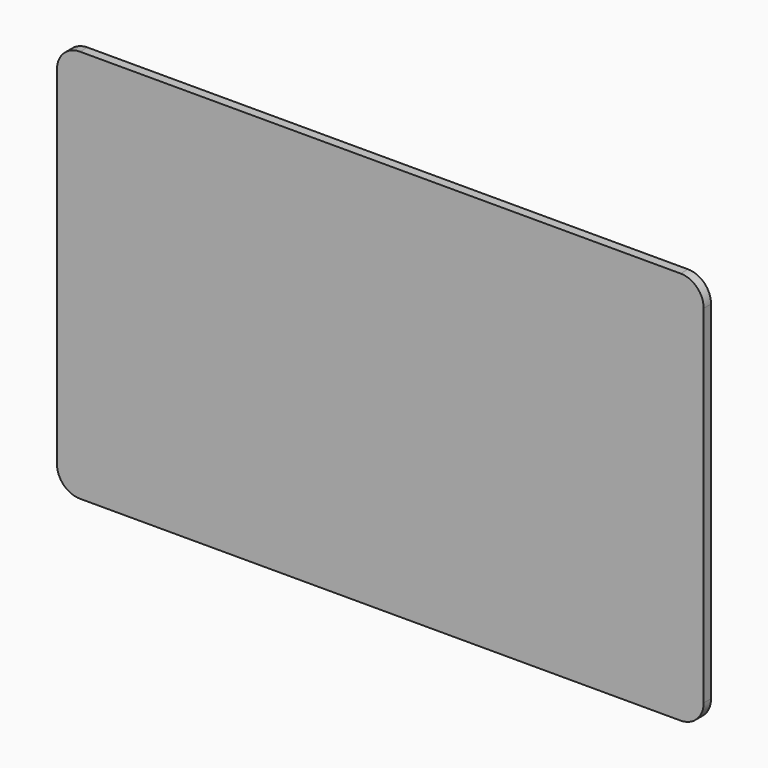
from build123d import *

# Parameters (mm, degrees)
F1_DEPTH = 3


# Not quite as in the source:
# - a feature names something its author has since deleted; it is built from what else it names


with BuildPart() as f1:
    # F0 (on Front) → F1 (new body)
    with BuildSketch(Plane.XZ):
        with BuildLine():
            ThreePointArc((105, 56.4), (102.8033008589, 61.7033008589), (97.5, 63.9))
            Line((97.5, 63.9), (-97.5, 63.9))
            ThreePointArc((-97.5, 63.9), (-102.8033008589, 61.7033008589), (-105, 56.4))
            Line((-105, 56.4), (-105, -56.4))
            ThreePointArc((-105, -56.4), (-102.8033008589, -61.7033008589), (-97.5, -63.9))
            Line((-97.5, -63.9), (97.5, -63.9))
            ThreePointArc((97.5, -63.9), (102.8033008589, -61.7033008589), (105, -56.4))
            Line((105, -56.4), (105, 56.4))
        make_face()
    extrude(amount=F1_DEPTH)


solid = f1.part
